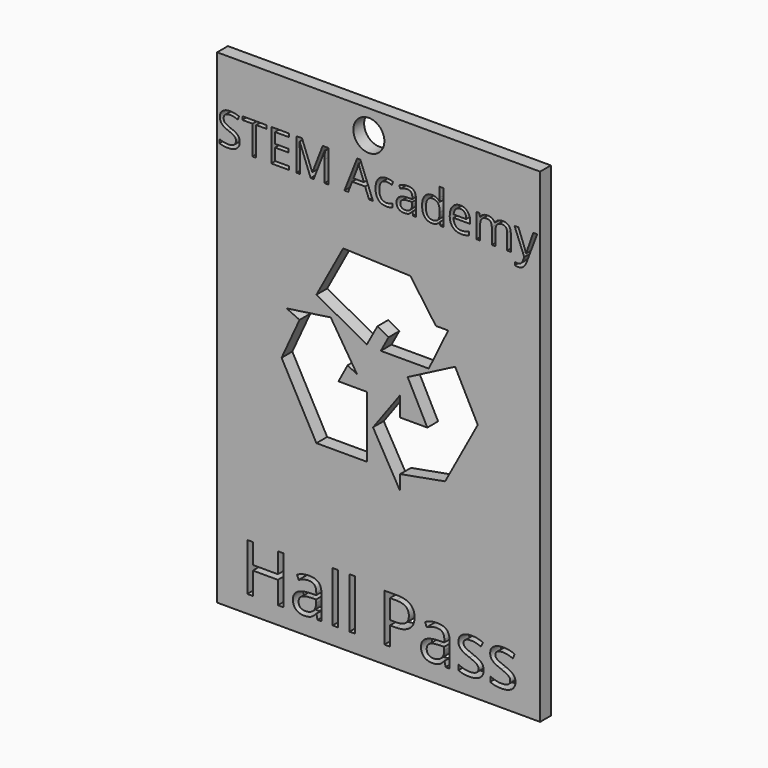
from build123d import *

# Parameters (mm, degrees)
F0_W         = 76.2
F0_H         = 114.3
F1_DEPTH     = 3.175
F2_TEXT_SIZE = 10.6457105435
F3_DEPTH     = 3.175
F4_R         = 3.6574396167
F5_DEPTH     = 25.4
F7_TEXT_SIZE = 15.705704896
F8_DEPTH     = 3.175
F9_DEPTH     = 3.175


# Not quite as in the source:
# - a length typed as a fraction of an inch, garbled in the dataset ("3 / 203.2 mm" for 3/8 in), is restored
# - Text() gives the source's letters only with a copy of the font that has no kerning and outlines rounded to 1/6400 em; it was checked with that copy


with BuildPart() as f1:
    # F0 (on Front) → F1 (new body)
    with BuildSketch(Plane.XZ):
        with Locations((14.6780908108, -4.3179224145)):
            Rectangle(F0_W, F0_H)
    extrude(amount=F1_DEPTH)

    # F2 (on face) → F3 (cut)
    with BuildSketch(Plane.XZ.offset(3.175)):
        with Locations((-23.4219091892, 33.9004247906)):
            Text('STEM Academy', F2_TEXT_SIZE, font='Open Sans', text_align=(TextAlign.LEFT, TextAlign.BOTTOM))
    extrude(amount=-F3_DEPTH, mode=Mode.SUBTRACT)

    # F4 (on face) → F5 (cut)
    with BuildSketch(Plane.XZ.offset(3.175)):
        with Locations((12.3756462708, 47.2001433372)):
            Circle(F4_R)
    extrude(amount=-F5_DEPTH, mode=Mode.SUBTRACT)

    # F7 (on face) → F8 (cut)
    with BuildSketch(Plane.XZ.offset(3.175)):
        with Locations((-17.8415272385, -57.3483668268)):
            Text('Hall Pass', F7_TEXT_SIZE, font='Open Sans', text_align=(TextAlign.LEFT, TextAlign.BOTTOM))
    extrude(amount=-F8_DEPTH, mode=Mode.SUBTRACT)

    # F6 (on face) → F9 (cut)
    with BuildSketch(Plane.XZ.offset(3.175)):
        Polygon((0, 10.0940861743), (11.9153214619, 3.6480934359), (14.3897524545, 8.2220422299), (20.1821103692, 18.9291294664), (22.1736263484, 21.2114807218), (6.3254878515, 21.7866561495), align=None)
        Polygon((20.1821103692, 18.9291294664), (14.3897524545, 8.2220422299), (17.0307168761, 6.7933239583), (15.1830259711, 3.3778948709), (26.512619108, 3.3778948709), (31.0926698148, 12.7776842564), (28.2000061125, 12.7776842564), (22.1736263484, 21.2114807218), align=None)
        Polygon((7.370766758, -2.1476997884), (9.6387593076, -3.3746464178), (3.3835824579, 6.4790365286), (-7.0279473571, 4.9764496461), (-3.979133442, 3.5781364422), (-8.220018819, -5.6684832089), (0, -20.7269471139), (11.9153214619, -20.7269471139), (11.9153214619, -6.201761526), (5.1966453902, -6.201761526), align=None)
        Polygon((13.3554264903, -13.1020396948), (19.7630748153, -24.2699107884), (19.7630748153, -20.7269471139), (30.3695034236, -18.7939796597), (30.8100651098, -17.9796079519), (26.1703524333, -8.9898039759), (19.7630748153, -8.9898039759), (19.7630748153, -4.3361145072), align=None)
        Polygon((26.1703524333, -8.9898039759), (30.8100651098, -17.9796079519), (38.0676683669, -4.5640365481), (32.729196218, 5.7796682231), (21.5306397568, 0), align=None)
    extrude(amount=-F9_DEPTH, mode=Mode.SUBTRACT)


solid = f1.part
